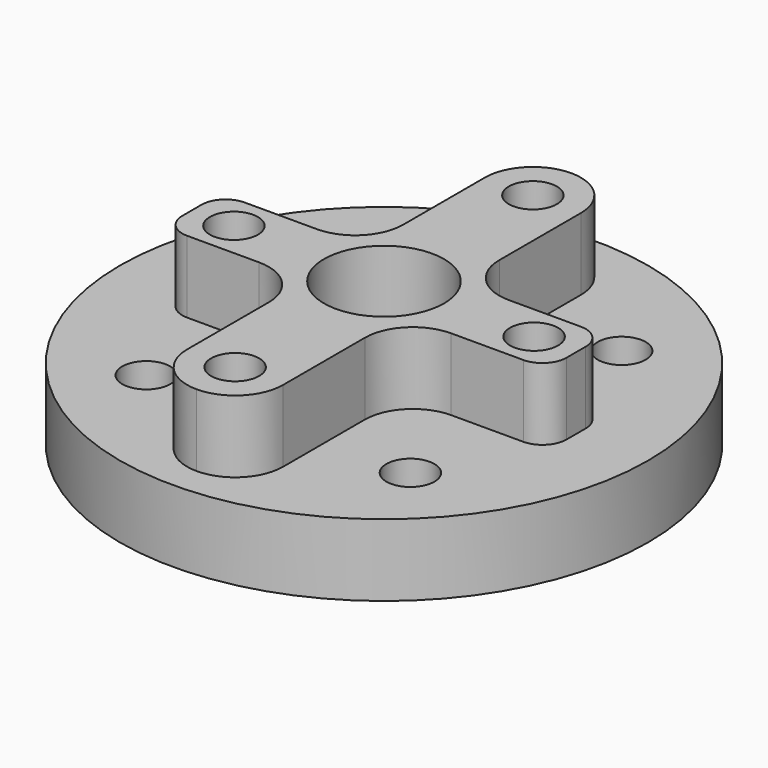
from build123d import *

# Parameters (mm, degrees)
F0_R     = 1
F0_R_2   = 2.5
F1_DEPTH = 3
F2_R     = 11
F2_R_2   = 1
F2_R_3   = 2.5
F3_DEPTH = 3


with BuildPart() as f1:
    # F0 (on Top) → F1 (new body)
    with BuildSketch(Plane.XY):
        with BuildLine():
            ThreePointArc((4, 1.5), (2.5857864376, 2.0857864376), (2, 3.5))
            Line((2, 3.5), (2, 7.75))
            ThreePointArc((2, 7.75), (1.4142135624, 9.1642135624), (0, 9.75))
            ThreePointArc((0, 9.75), (-1.4142135624, 9.1642135624), (-2, 7.75))
            Line((-2, 7.75), (-2, 3.5))
            ThreePointArc((-2, 3.5), (-2.5857864376, 2.0857864376), (-4, 1.5))
            Line((-4, 1.5), (-7, 1.5))
            ThreePointArc((-7, 1.5), (-7.7071067812, 1.2071067812), (-8, 0.5))
            Line((-8, 0.5), (-8, -0.5))
            ThreePointArc((-8, -0.5), (-7.7071067812, -1.2071067812), (-7, -1.5))
            Line((-7, -1.5), (-4, -1.5))
            ThreePointArc((-4, -1.5), (-2.5857864376, -2.0857864376), (-2, -3.5))
            Line((-2, -3.5), (-2, -7.75))
            ThreePointArc((-2, -7.75), (-1.4142135624, -9.1642135624), (0, -9.75))
            ThreePointArc((0, -9.75), (1.4142135624, -9.1642135624), (2, -7.75))
            Line((2, -7.75), (2, -3.5))
            ThreePointArc((2, -3.5), (2.5857864376, -2.0857864376), (4, -1.5))
            Line((4, -1.5), (7, -1.5))
            ThreePointArc((7, -1.5), (7.7071067812, -1.2071067812), (8, -0.5))
            Line((8, -0.5), (8, 0.5))
            ThreePointArc((8, 0.5), (7.7071067812, 1.2071067812), (7, 1.5))
            Line((7, 1.5), (4, 1.5))
        make_face()
        with Locations((0, -7.75)):
            Circle(F0_R, mode=Mode.SUBTRACT)
        with Locations((-6.25, 0)):
            Circle(F0_R, mode=Mode.SUBTRACT)
        Circle(F0_R_2, mode=Mode.SUBTRACT)
        with Locations((6.25, 0)):
            Circle(F0_R, mode=Mode.SUBTRACT)
        with Locations((0, 7.75)):
            Circle(F0_R, mode=Mode.SUBTRACT)
    extrude(amount=F1_DEPTH)

    # F2 (on face) → F3 (join)
    with BuildSketch(Plane(origin=(0, 0, 0), x_dir=(1, 0, 0), z_dir=(0, 0, -1))):
        Circle(F2_R)
        with Locations((-5.5, -5.5)):
            Circle(F2_R_2, mode=Mode.SUBTRACT)
        with Locations((5.5, -5.5)):
            Circle(F2_R_2, mode=Mode.SUBTRACT)
        with Locations((-5.5, 5.5)):
            Circle(F2_R_2, mode=Mode.SUBTRACT)
        with BuildLine():
            ThreePointArc((-2, 7.75), (0, 9.75), (2, 7.75))
            Line((2, 7.75), (2, 3.5))
            ThreePointArc((2, 3.5), (2.5857864376, 2.0857864376), (4, 1.5))
            Line((4, 1.5), (7, 1.5))
            ThreePointArc((7, 1.5), (7.7071067812, 1.2071067812), (8, 0.5))
            Line((8, 0.5), (8, -0.5))
            ThreePointArc((8, -0.5), (7.7071067812, -1.2071067812), (7, -1.5))
            Line((7, -1.5), (4, -1.5))
            ThreePointArc((4, -1.5), (2.5857864376, -2.0857864376), (2, -3.5))
            Line((2, -3.5), (2, -7.75))
            ThreePointArc((2, -7.75), (0, -9.75), (-2, -7.75))
            Line((-2, -7.75), (-2, -3.5))
            ThreePointArc((-2, -3.5), (-2.5857864376, -2.0857864376), (-4, -1.5))
            Line((-4, -1.5), (-7, -1.5))
            ThreePointArc((-7, -1.5), (-7.7071067812, -1.2071067812), (-8, -0.5))
            Line((-8, -0.5), (-8, 0.5))
            ThreePointArc((-8, 0.5), (-7.7071067812, 1.2071067812), (-7, 1.5))
            Line((-7, 1.5), (-4, 1.5))
            ThreePointArc((-4, 1.5), (-2.5857864376, 2.0857864376), (-2, 3.5))
            Line((-2, 3.5), (-2, 7.75))
        make_face(mode=Mode.SUBTRACT)
        with Locations((5.5, 5.5)):
            Circle(F2_R_2, mode=Mode.SUBTRACT)
        with BuildLine():
            Line((2, 3.5), (2, 7.75))
            ThreePointArc((2, 7.75), (0, 9.75), (-2, 7.75))
            Line((-2, 7.75), (-2, 3.5))
            ThreePointArc((-2, 3.5), (-2.5857864376, 2.0857864376), (-4, 1.5))
            Line((-4, 1.5), (-7, 1.5))
            ThreePointArc((-7, 1.5), (-7.7071067812, 1.2071067812), (-8, 0.5))
            Line((-8, 0.5), (-8, -0.5))
            ThreePointArc((-8, -0.5), (-7.7071067812, -1.2071067812), (-7, -1.5))
            Line((-7, -1.5), (-4, -1.5))
            ThreePointArc((-4, -1.5), (-2.5857864376, -2.0857864376), (-2, -3.5))
            Line((-2, -3.5), (-2, -7.75))
            ThreePointArc((-2, -7.75), (0, -9.75), (2, -7.75))
            Line((2, -7.75), (2, -3.5))
            ThreePointArc((2, -3.5), (2.5857864376, -2.0857864376), (4, -1.5))
            Line((4, -1.5), (7, -1.5))
            ThreePointArc((7, -1.5), (7.7071067812, -1.2071067812), (8, -0.5))
            Line((8, -0.5), (8, 0.5))
            ThreePointArc((8, 0.5), (7.7071067812, 1.2071067812), (7, 1.5))
            Line((7, 1.5), (4, 1.5))
            ThreePointArc((4, 1.5), (2.5857864376, 2.0857864376), (2, 3.5))
        make_face()
        with Locations((0, -7.75)):
            Circle(F2_R_2, mode=Mode.SUBTRACT)
        with Locations((-6.25, 0)):
            Circle(F2_R_2, mode=Mode.SUBTRACT)
        Circle(F2_R_3, mode=Mode.SUBTRACT)
        with Locations((6.25, 0)):
            Circle(F2_R_2, mode=Mode.SUBTRACT)
        with Locations((0, 7.75)):
            Circle(F2_R_2, mode=Mode.SUBTRACT)
    extrude(amount=F3_DEPTH)


solid = f1.part
